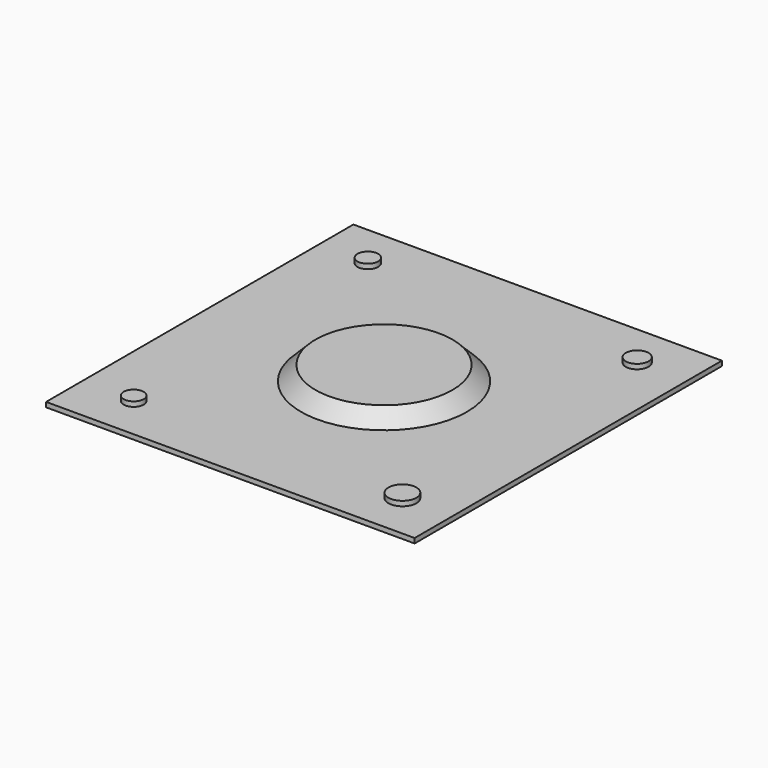
from build123d import *

# Parameters (mm, degrees)
F1_R     = 24.1613499239
F2_DEPTH = 4
F0_W     = 76.2569829822
F0_H     = 79.4832408428
F3_DEPTH = 1
F4_R     = 2.0739165502
F5_DEPTH = 1
F6_R     = 2.8886313869
F6_R_2   = 2.3646284302
F6_R_3   = 2.1352299697
F7_DEPTH = 1


# Not quite as in the source:
# - a fillet or chamfer that OpenCascade refuses, or shapes differently, is made with other operations: its cross-section is extruded or revolved along the edge and cut away or added


with BuildPart() as f2:
    # F1 (on face) → F2 (new body)
    with BuildSketch(Plane.XY):
        Circle(F1_R)
    extrude(amount=F2_DEPTH)

    # F0 (on Top) → F3 (join)
    with BuildSketch(Plane.XY):
        Rectangle(F0_W, F0_H)
    extrude(amount=F3_DEPTH)

    # F4 (on face) → F5 (join)
    with BuildSketch(Plane.XY.offset(1)):
        with Locations((-27.2765364498, -30.6494422257)):
            Circle(F4_R)
    extrude(amount=F5_DEPTH)

    # F6 (on face) → F7 (join)
    with BuildSketch(Plane.XY.offset(1)):
        with Locations((27.8631281108, -30.0628505647)):
            Circle(F6_R)
        with Locations((27.8631281108, 30.6494422257)):
            Circle(F6_R_2)
        with Locations((-27.8631299734, 30.6494422257)):
            Circle(F6_R_3)
    extrude(amount=F7_DEPTH)

    # F8: chamfer of 10 on 1 edges, made by hand


with BuildPart() as f8_tool2:
    # F8_s3 → F8_t4 (revolve)
    with BuildSketch(Plane.XZ):
        with BuildLine():
            Line((24.4441926363, -6.2828427125), (13.8785072114, 4.2828427125))
            Line((13.8785072114, 4.2828427125), (13.8785072114, 4.4828427125))
            ThreePointArc((13.8785072114, 4.4828427125), (19.0199285676, 4.2), (24.1613499239, 4.2))
            Line((24.1613499239, 4.2), (24.3613499239, 4))
            ThreePointArc((24.3613499239, 4), (24.3613499239, -1.1414213562), (24.6441926363, -6.2828427125))
            Line((24.6441926363, -6.2828427125), (24.4441926363, -6.2828427125))
        make_face()
    revolve(axis=Axis((0, 0, 4), (0, 0, 1)))

    split(bisect_by=Plane.XY.offset(1), keep=Keep.TOP)


with BuildPart() as f2_1:
    add(f2.part)

    # F8_t1: cut F8_tool2
    add(f8_tool2.part, mode=Mode.SUBTRACT)


solid = f2_1.part
